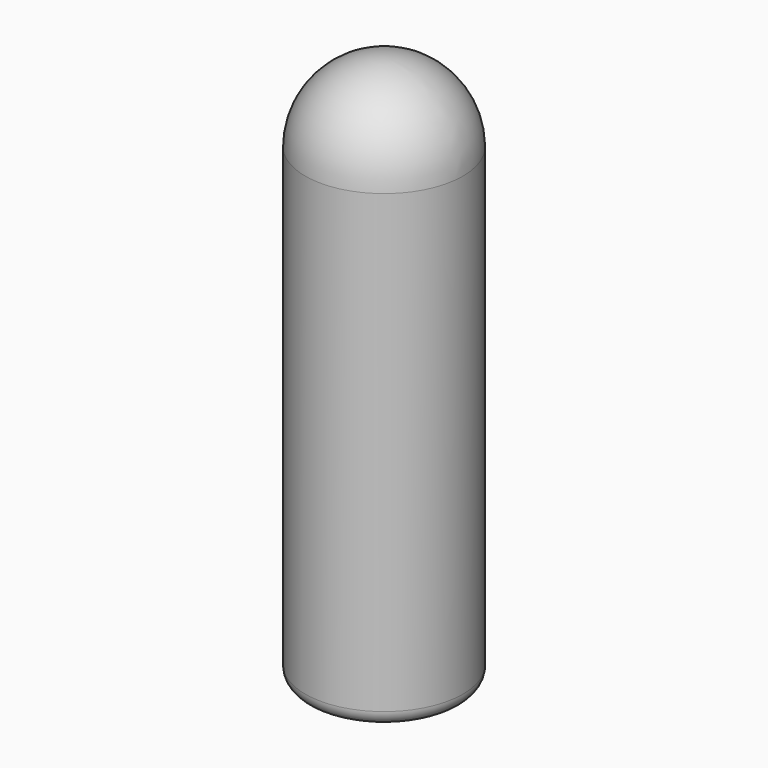
from build123d import *

# Parameters (mm, degrees)
F2_T = -1.016


# Not quite as in the source:
# - a shell that OpenCascade refuses in one call is made with other operations: the cavity is built on its own and cut out


with BuildPart() as f1:
    # F0 (on Front) → F1 (revolve)
    with BuildSketch(Plane.XZ):
        with BuildLine():
            Line((0, 109.22), (0, 0))
            Line((0, 0), (12.7, 0))
            ThreePointArc((12.7, 0), (14.8013799323, 0.8704200677), (15.6718, 2.9718))
            Line((15.6718, 2.9718), (15.6718, 93.5482))
            ThreePointArc((15.6718, 93.5482), (11.0816360534, 104.6298360534), (0, 109.22))
        make_face()
    revolve(axis=Axis((0, 0, 54.61), (0, 0, 1)))

    # F2: a shell. OpenCascade refuses it in one call, so the cavity is built on its own and cut out:
    # the body offset inwards by the wall thickness, plus a prism from it out through each open face.
    f2_core = offset(f1.part, amount=F2_T, mode=Mode.PRIVATE)
    f2_exits = [f2_core.faces().sort_by_distance(p)[0] for p in [
        (0, 0, 1.016),
    ]]
    add(f2_core, mode=Mode.SUBTRACT)
    extrude(f2_exits, amount=-F2_T, mode=Mode.SUBTRACT)


solid = f1.part
